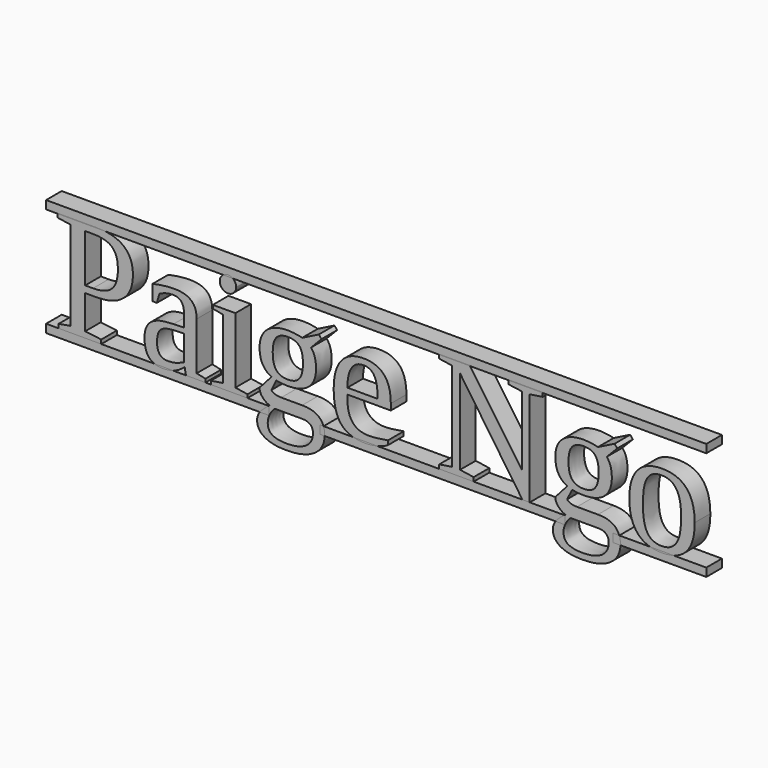
from build123d import *

# Parameters (mm, degrees)
F0_TEXT_SIZE = 23.7063377412
F1_DEPTH     = 3
F2_W         = 34.2256866975
F2_H         = 1.27
F2_W_2       = 37.5693861278
F2_W_3       = 14.307551944
F3_DEPTH     = 3
F5_DEPTH     = 3


# Not quite as in the source:
# - Text() gives the source's letters only with a copy of the font that has no kerning and outlines rounded to 1/6400 em; it was checked with that copy


with BuildPart() as f1:
    # F0 (on Front) → F1 (new body)
    with BuildSketch(Plane.XZ):
        with Locations((-49.8911338358, 0)):
            Text('Paige Ngo', F0_TEXT_SIZE, font='Tinos', text_align=(TextAlign.LEFT, TextAlign.BOTTOM))
    extrude(amount=F1_DEPTH)

    # F2 (on Front) → F3 (join)
    with BuildSketch(Plane.XZ):
        with Locations((-33.874733277, -0.635)):
            Rectangle(F2_W, F2_H)
        with Locations((9.8889669462, -0.635)):
            Rectangle(F2_W_2, F2_H)
        with Locations((43.2514440833, -0.635)):
            Rectangle(F2_W_3, F2_H)
    extrude(amount=F3_DEPTH)

    # F4 (on Front) → F5 (join)
    with BuildSketch(Plane.XZ):
        Polygon((50.4052200553, 16.7180128007), (-50.9875766258, 16.7180128007), (-50.9875766258, 15.4480128007), (-48.969142139, 15.4480128007), (-41.9379584491, 15.4480128007), (50.4052200553, 15.4480128007), align=None)
    extrude(amount=F5_DEPTH)


solid = f1.part
